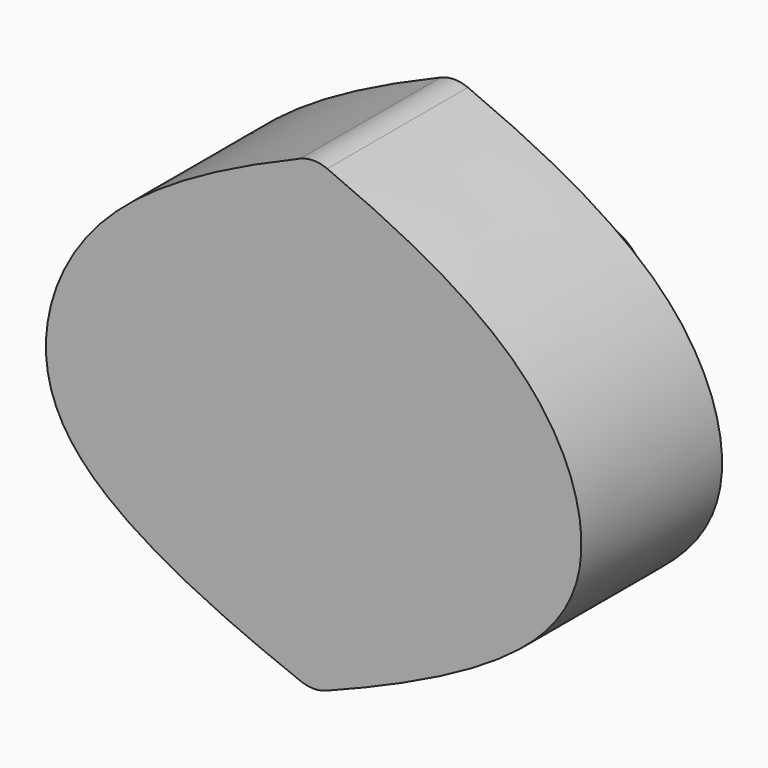
from build123d import *

# Parameters (mm, degrees)
F1_DEPTH = 25
F2_R     = 7.5
F3_DEPTH = 25
F4_R     = 5


with BuildPart() as f1:
    # F0 (on Front) → F1 (new body)
    with BuildSketch(Plane.XZ):
        with BuildLine():
            add(Edge.make_bspline(
                [(0, 35.3876687586), (13.8926569286, 29.7244304014), (32.1401882045, 19.7182221568), (39.9630337201, 0.1220754807), (34.1200278266, -16.2486022664), (15.2266629868, -25.7030703609), (0, -31.4665324986)],
                knots=[0, 0, 0, 0, 0.2989563536, 0.5089024667, 0.6954830611, 1, 1, 1, 1], degree=3))
            add(Edge.make_bspline(
                [(0, 35.3876687586), (-13.8926569286, 29.7244304014), (-32.1401882045, 19.7182221568), (-39.9630337201, 0.1220754807), (-34.1200278266, -16.2486022664), (-15.2266629868, -25.7030703609), (0, -31.4665324986)],
                knots=[0, 0, 0, 0, 0.2989563536, 0.5089024667, 0.6954830611, 1, 1, 1, 1], degree=3))
        make_face()
    extrude(amount=F1_DEPTH)

    # F2 (on face) → F3 (join)
    with BuildSketch(Plane(origin=(0, 0, 0), x_dir=(-1, 0, 0), z_dir=(0, 1, 0))):
        Circle(F2_R)
    extrude(amount=F3_DEPTH)

    # F4
    f4_edges = [f1.edges().sort_by_distance(p)[0] for p in [
        (0, -12.5, 35.387669),
        (0, -12.5, -31.466532),
    ]]
    fillet(f4_edges, radius=F4_R)


solid = f1.part
